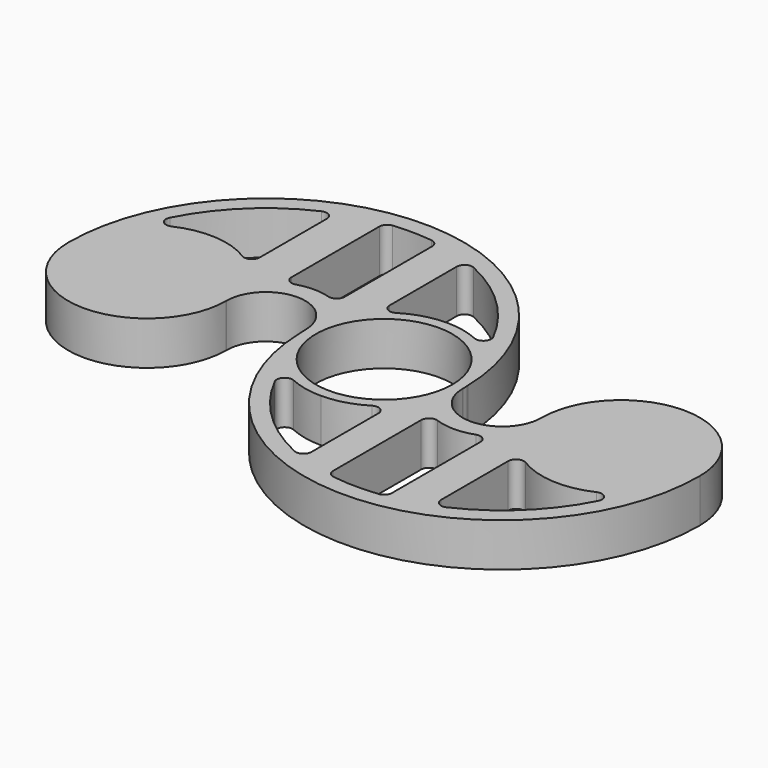
from build123d import *

# Parameters (mm, degrees)
F0_R        = 10.9855
F0_R_2      = 10.989999991
F1_DEPTH    = 7
F2_T1_DEPTH = 7
F2_T3_DEPTH = 7.1579854221
F2_T5_DEPTH = 7.1579856015
F2_T7_DEPTH = 7.1579856772
F3_R        = 1.27


# Not quite as in the source:
# - a fillet or chamfer that OpenCascade refuses, or shapes differently, is made with other operations: its cross-section is extruded or revolved along the edge and cut away or added
# - a feature names something its author has since deleted; it is built from what else it names


with BuildPart() as f1:
    # F0 (on Top) → F1 (new body)
    with BuildSketch(Plane.XY):
        with BuildLine():
            ThreePointArc((0.0122500747, -12.699994092), (8.9845861326, -8.9759240207), (12.7, 0))
            ThreePointArc((12.7, 0), (11.6341942626, 5.0926931834), (8.6156655339, 9.3306113095))
            ThreePointArc((8.6156655339, 9.3306113095), (4.6312435718, 11.8254633304), (0.0122500747, 12.699994092))
            ThreePointArc((0.0122500747, 12.699994092), (-4.6067434223, 11.8254633304), (-8.5911653844, 9.3306113095))
            ThreePointArc((-8.5911653844, 9.3306113095), (-11.6096941131, 5.0926931834), (-12.6754998505, 0))
            ThreePointArc((-12.6754998505, 0), (-11.6096941131, -5.0926931834), (-8.5911653844, -9.3306113095))
            ThreePointArc((-8.5911653844, -9.3306113095), (-4.6067434223, -11.8254633304), (0.0122500747, -12.699994092))
        make_face()
        with Locations((0.0245001495, 0)):
            Circle(F0_R, mode=Mode.SUBTRACT)
        with BuildLine():
            ThreePointArc((12.7245001495, 0), (12.716207726, 0.4588668575), (12.6913412845, 0.9171344838))
            ThreePointArc((12.6913412845, 0.9171344838), (12.6989837582, 0.4585985212), (12.7, 0))
            ThreePointArc((12.7, 0), (8.9845861326, -8.9759240207), (0.0122500747, -12.699994092))
            ThreePointArc((0.0122500747, -12.699994092), (4.6443350463, -11.8299250009), (8.6401656833, -9.3306113095))
            ThreePointArc((8.6401656833, -9.3306113095), (10.2086695664, -7.5876671836), (11.4300151579, -5.586074417))
            ThreePointArc((11.4300151579, -5.586074417), (12.3868415398, -2.9090402797), (12.7242073512, -0.086237983))
            ThreePointArc((12.7242073512, -0.086237983), (12.7242070748, -0.0431184935), (12.7245001495, 0))
        make_face()
        with BuildLine():
            ThreePointArc((25.4002735579, -0.086237983), (19.0622404546, -6.4027075191), (12.7242073512, -0.086237983))
            ThreePointArc((12.7242073512, -0.086237983), (12.3868415398, -2.9090402797), (11.4300151579, -5.586074417))
            ThreePointArc((11.4300151579, -5.586074417), (12.5867658694, -6.9038365057), (13.9769937331, -7.9724035921))
            ThreePointArc((13.9769937331, -7.9724035921), (18.7426985376, -9.3370960194), (23.5084033421, -7.9724035921))
            ThreePointArc((23.5084033421, -7.9724035921), (25.1435205419, -6.6655071902), (26.4326717576, -5.0163632895))
            ThreePointArc((26.4326717576, -5.0163632895), (25.6695984826, -2.6029975888), (25.4002735579, -0.086237983))
        make_face()
        with BuildLine():
            ThreePointArc((46.7156462935, -9.3306113095), (49.7341750222, -5.0926931834), (50.7999807596, 0))
            ThreePointArc((50.7999807596, 0), (38.0999807596, 12.7), (25.3999807596, 0))
            ThreePointArc((25.3999807596, 0), (25.4002738343, -0.0431184935), (25.4002735579, -0.086237983))
            ThreePointArc((25.4002735579, -0.086237983), (25.6695984826, -2.6029975888), (26.4326717576, -5.0163632895))
            ThreePointArc((26.4326717576, -5.0163632895), (27.7316179187, -7.3339656394), (29.4843152258, -9.3306113095))
            ThreePointArc((29.4843152258, -9.3306113095), (38.0999807596, -12.7), (46.7156462935, -9.3306113095))
        make_face()
        with Locations((38.0999807596, 0)):
            Circle(F0_R_2, mode=Mode.SUBTRACT)
        with BuildLine():
            ThreePointArc((-8.5801649897, -9.3632669913), (-11.43210855, -5.5314459322), (-12.666841135, -0.9171344838))
            ThreePointArc((-12.666841135, -0.9171344838), (19.5208281328, -31.8937955885), (50.7999807596, 0))
            ThreePointArc((50.7999807596, 0), (49.7341750222, -5.0926931834), (46.7156462935, -9.3306113095))
            ThreePointArc((46.7156462935, -9.3306113095), (40.1099512813, -20.2359805679), (29.4843152258, -27.2828340268))
            ThreePointArc((29.4843152258, -27.2828340268), (26.5384433366, -28.2337157759), (23.5084033421, -28.8671152702))
            ThreePointArc((23.5084033421, -28.8671152702), (18.7383474141, -29.2061036376), (13.9769937331, -28.7612915499))
            ThreePointArc((13.9769937331, -28.7612915499), (11.2734206382, -28.1489774328), (8.6401656833, -27.2828340268))
            ThreePointArc((8.6401656833, -27.2828340268), (-1.9735358373, -20.2484070502), (-8.5801649897, -9.3632669913))
        make_face()
        with BuildLine():
            ThreePointArc((-11.4055150084, 5.586074417), (-12.3623413903, 2.9090402797), (-12.6997072018, 0.086237983))
            ThreePointArc((-12.6997072018, 0.086237983), (-12.6997069253, 0.0431184935), (-12.7, 0))
            ThreePointArc((-12.7, 0), (-12.6917075765, -0.4588668575), (-12.666841135, -0.9171344838))
            ThreePointArc((-12.666841135, -0.9171344838), (-12.6744836087, -0.4585985212), (-12.6754998505, 0))
            ThreePointArc((-12.6754998505, 0), (-11.6096941131, 5.0926931834), (-8.5911653844, 9.3306113095))
            Line((-8.5911653844, 9.3306113095), (-8.5911653844, 9.3531747198))
            ThreePointArc((-8.5911653844, 9.3531747198), (-10.1742109205, 7.6010152049), (-11.4055150084, 5.586074417))
        make_face()
        with BuildLine():
            ThreePointArc((-22.9900462212, 8.2591606127), (-24.9149898439, 6.8653148973), (-26.4081716081, 5.0163632895))
            ThreePointArc((-26.4081716081, 5.0163632895), (-25.6450983331, 2.6029975888), (-25.3757734084, 0.086237983))
            ThreePointArc((-25.3757734084, 0.086237983), (-19.0377403051, 6.4027075191), (-12.6997072018, 0.086237983))
            ThreePointArc((-12.6997072018, 0.086237983), (-12.3623413903, 2.9090402797), (-11.4055150084, 5.586074417))
            ThreePointArc((-11.4055150084, 5.586074417), (-12.773731355, 7.0957580254), (-14.446350555, 8.2591606127))
            ThreePointArc((-14.446350555, 8.2591606127), (-18.7181983881, 9.3370960194), (-22.9900462212, 8.2591606127))
        make_face()
        with BuildLine():
            ThreePointArc((-25.3757734084, 0.086237983), (-25.6450983331, 2.6029975888), (-26.4081716081, 5.0163632895))
            ThreePointArc((-26.4081716081, 5.0163632895), (-27.7071177693, 7.3339656394), (-29.4598150763, 9.3306113095))
            ThreePointArc((-29.4598150763, 9.3306113095), (-38.0754806101, 12.7), (-46.691146144, 9.3306113095))
            ThreePointArc((-46.691146144, 9.3306113095), (-49.7096748727, 5.0926931834), (-50.7754806101, 0))
            ThreePointArc((-50.7754806101, 0), (-38.0754806101, -12.7), (-25.3754806101, 0))
            ThreePointArc((-25.3754806101, 0), (-25.3757736848, 0.0431184935), (-25.3757734084, 0.086237983))
        make_face()
        with Locations((-38.0754806101, 0)):
            Circle(F0_R_2, mode=Mode.SUBTRACT)
        with BuildLine():
            ThreePointArc((-8.5911653844, -9.3306113095), (-8.5856700083, -9.3469407745), (-8.5801649897, -9.3632669913))
            ThreePointArc((-8.5801649897, -9.3632669913), (-4.5973610293, -11.8386769348), (0.0122500747, -12.699994092))
            ThreePointArc((0.0122500747, -12.699994092), (-4.6067434223, -11.8254633304), (-8.5911653844, -9.3306113095))
        make_face()
        with BuildLine():
            ThreePointArc((-12.6754998505, 0), (-12.6744836087, -0.4585985212), (-12.666841135, -0.9171344838))
            ThreePointArc((-12.666841135, -0.9171344838), (-11.43210855, -5.5314459322), (-8.5801649897, -9.3632669913))
            ThreePointArc((-8.5801649897, -9.3632669913), (-8.5856700083, -9.3469407745), (-8.5911653844, -9.3306113095))
            ThreePointArc((-8.5911653844, -9.3306113095), (-11.6096941131, -5.0926931834), (-12.6754998505, 0))
        make_face()
        with BuildLine():
            ThreePointArc((12.7, 0), (12.6989837582, 0.4585985212), (12.6913412845, 0.9171344838))
            ThreePointArc((12.6913412845, 0.9171344838), (11.4566086995, 5.5314459323), (8.6046651392, 9.3632669913))
            ThreePointArc((8.6046651392, 9.3632669913), (8.6101701578, 9.3469407745), (8.6156655339, 9.3306113095))
            ThreePointArc((8.6156655339, 9.3306113095), (11.6341942626, 5.0926931834), (12.7, 0))
        make_face()
        with BuildLine():
            ThreePointArc((8.6156655339, 9.3306113095), (8.6101701578, 9.3469407745), (8.6046651392, 9.3632669913))
            ThreePointArc((8.6046651392, 9.3632669913), (4.6218611788, 11.8386769348), (0.0122500747, 12.699994092))
            ThreePointArc((0.0122500747, 12.699994092), (4.6312435718, 11.8254633304), (8.6156655339, 9.3306113095))
        make_face()
        with BuildLine():
            ThreePointArc((-50.7754806101, 0), (-49.7096748727, 5.0926931834), (-46.691146144, 9.3306113095))
            ThreePointArc((-46.691146144, 9.3306113095), (-40.0854511318, 20.2359805679), (-29.4598150763, 27.2828340268))
            ThreePointArc((-29.4598150763, 27.2828340268), (-26.2724748955, 28.2966277505), (-22.9900462212, 28.9389494304))
            ThreePointArc((-22.9900462212, 28.9389494304), (-18.7147163655, 29.2061132739), (-14.446350555, 28.8443464952))
            ThreePointArc((-14.446350555, 28.8443464952), (-11.4778445606, 28.2113948339), (-8.5911653844, 27.2734508175))
            ThreePointArc((-8.5911653844, 27.2734508175), (2.0071231414, 20.238946653), (8.6046651392, 9.3632669913))
            ThreePointArc((8.6046651392, 9.3632669913), (11.4566086995, 5.5314459323), (12.6913412845, 0.9171344838))
            ThreePointArc((12.6913412845, 0.9171344838), (-19.4963279834, 31.8937955885), (-50.7754806101, 0))
        make_face()
        with BuildLine():
            Line((-14.446350555, 28.8443464952), (-14.446350555, 8.2591606127))
            ThreePointArc((-14.446350555, 8.2591606127), (-12.773731355, 7.0957580254), (-11.4055150084, 5.586074417))
            ThreePointArc((-11.4055150084, 5.586074417), (-10.1742109205, 7.6010152049), (-8.5911653844, 9.3531747198))
            Line((-8.5911653844, 9.3531747198), (-8.5911653844, 27.2734508175))
            ThreePointArc((-8.5911653844, 27.2734508175), (-11.4778445606, 28.2113948339), (-14.446350555, 28.8443464952))
        make_face()
        with BuildLine():
            ThreePointArc((-29.4598150763, 9.3306113095), (-27.7071177693, 7.3339656394), (-26.4081716081, 5.0163632895))
            ThreePointArc((-26.4081716081, 5.0163632895), (-24.9149898439, 6.8653148973), (-22.9900462212, 8.2591606127))
            Line((-22.9900462212, 8.2591606127), (-22.9900462212, 28.9389494304))
            ThreePointArc((-22.9900462212, 28.9389494304), (-26.2724748955, 28.2966277505), (-29.4598150763, 27.2828340268))
            Line((-29.4598150763, 27.2828340268), (-29.4598150763, 9.3306113095))
        make_face()
        with BuildLine():
            Line((8.6401656833, -9.3306113095), (8.6401656833, -27.2828340268))
            ThreePointArc((8.6401656833, -27.2828340268), (11.2734206382, -28.1489774328), (13.9769937331, -28.7612915499))
            Line((13.9769937331, -28.7612915499), (13.9769937331, -7.9724035921))
            ThreePointArc((13.9769937331, -7.9724035921), (12.5867658694, -6.9038365057), (11.4300151579, -5.586074417))
            ThreePointArc((11.4300151579, -5.586074417), (10.2086695664, -7.5876671836), (8.6401656833, -9.3306113095))
        make_face()
        with BuildLine():
            Line((29.4843152258, -27.2828340268), (29.4843152258, -9.3306113095))
            ThreePointArc((29.4843152258, -9.3306113095), (27.7316179187, -7.3339656394), (26.4326717576, -5.0163632895))
            ThreePointArc((26.4326717576, -5.0163632895), (25.1435205419, -6.6655071902), (23.5084033421, -7.9724035921))
            Line((23.5084033421, -7.9724035921), (23.5084033421, -28.8671152702))
            ThreePointArc((23.5084033421, -28.8671152702), (26.5384433366, -28.2337157759), (29.4843152258, -27.2828340268))
        make_face()
        with Locations((-38.0754806101, 0)):
            Circle(F0_R_2)
        with Locations((38.0999807596, 0)):
            Circle(F0_R_2)
    extrude(amount=F1_DEPTH)

    # F2: fillet of radius 5.08 on 9 edges, made by hand

    # F2_s2 → F2_t1 (join)
    with BuildSketch(Plane.XY):
        with BuildLine():
            ThreePointArc((-50.7755312412, 0.0104518732), (-50.7754943345, 0.0004688293), (-50.7754770463, -0.0095142678))
            ThreePointArc((-50.7754770463, -0.0095142678), (-50.7754797192, -0.0047571342), (-50.7754806101, 0))
            ThreePointArc((-50.7754806101, 0), (-50.7755063559, 0.0052259345), (-50.7755312412, 0.0104518732))
        make_face()
        with BuildLine():
            ThreePointArc((-12.6731476592, -0.8254261976), (-12.6677935321, -0.9217143052), (-12.6642681854, -1.018086699))
            ThreePointArc((-12.6642681854, -1.018086699), (-12.6655948117, -0.9676116147), (-12.666841135, -0.9171344838))
            ThreePointArc((-12.666841135, -0.9171344838), (-12.6700773725, -0.8712860467), (-12.6731476592, -0.8254261976))
        make_face()
        with BuildLine():
            ThreePointArc((12.6976478087, 0.8254261976), (12.6922936816, 0.9217143052), (12.6887683349, 1.018086699))
            ThreePointArc((12.6887683349, 1.018086699), (12.6900949612, 0.9676116147), (12.6913412845, 0.9171344838))
            ThreePointArc((12.6913412845, 0.9171344838), (12.694577522, 0.8712860467), (12.6976478087, 0.8254261976))
        make_face()
        with BuildLine():
            ThreePointArc((50.8000313907, -0.0104518732), (50.799994484, -0.0004688294), (50.7999771958, 0.0095142678))
            ThreePointArc((50.7999771958, 0.0095142678), (50.7999798687, 0.0047571342), (50.7999807596, 0))
            ThreePointArc((50.7999807596, 0), (50.8000065054, -0.0052259345), (50.8000313907, -0.0104518732))
        make_face()
    extrude(amount=F2_T1_DEPTH)

    # F2_s4 → F2_t3 (cut)
    with BuildSketch(Plane.XY.offset(-0.0789927111)):
        with BuildLine():
            ThreePointArc((-12.6998402645, 0.0182342924), (-12.6999615812, -0.0066812361), (-12.6999606939, -0.03159706))
            ThreePointArc((-12.6999606939, -0.03159706), (-12.6999901735, -0.0157985422), (-12.7, 0))
            ThreePointArc((-12.7, 0), (-12.6999135747, 0.0091170887), (-12.6998402645, 0.0182342924))
        make_face()
    extrude(amount=F2_T3_DEPTH, mode=Mode.SUBTRACT)

    # F2_s6 → F2_t5 (cut)
    with BuildSketch(Plane.XY.offset(-0.0789928007)):
        with BuildLine():
            ThreePointArc((-25.3756403458, 0.0182342804), (-25.375519029, -0.0066812601), (-25.3755199164, -0.0315970958))
            ThreePointArc((-25.3755199164, -0.0315970958), (-25.3754904367, -0.0157985601), (-25.3754806101, 0))
            ThreePointArc((-25.3754806101, 0), (-25.3755670356, 0.0091170828), (-25.3756403458, 0.0182342804))
        make_face()
        with BuildLine():
            ThreePointArc((25.4000200658, 0.0315970958), (25.4000191785, 0.0066812601), (25.4001404953, -0.0182342804))
            ThreePointArc((25.4001404953, -0.0182342804), (25.4000671851, -0.0091170828), (25.3999807596, 0))
            ThreePointArc((25.3999807596, 0), (25.3999905862, 0.0157985601), (25.4000200658, 0.0315970958))
        make_face()
    extrude(amount=F2_T5_DEPTH, mode=Mode.SUBTRACT)

    # F2_s8 → F2_t7 (cut)
    with BuildSketch(Plane.XY.offset(-0.0789928386)):
        with BuildLine():
            ThreePointArc((12.7243404138, -0.0182342754), (12.7244617306, 0.0066812701), (12.7244608432, 0.031597111))
            ThreePointArc((12.7244608432, 0.031597111), (12.7244903229, 0.0157985677), (12.7245001495, 0))
            ThreePointArc((12.7245001495, 0), (12.724413724, -0.0091170802), (12.7243404138, -0.0182342754))
        make_face()
    extrude(amount=F2_T7_DEPTH, mode=Mode.SUBTRACT)

    # F3
    f3_edges = [f1.edges().sort_by_distance(p)[0] for p in [
        (29.484315, -27.282834, 3.5),
        (29.484315, -9.330611, 3.5),
        (46.715646, -9.330611, 3.5),
        (23.508403, -7.972404, 3.5),
        (13.976994, -7.972404, 3.5),
        (23.508403, -28.867115, 3.5),
        (13.976994, -28.761292, 3.5),
        (8.640166, -27.282834, 3.5),
        (8.640166, -9.330611, 3.5),
        (-8.580165, -9.363267, 3.5),
        (-22.990046, 28.938949, 3.5),
        (-8.591165, 27.273451, 3.5),
        (8.604665, 9.363267, 3.5),
        (-8.591165, 9.330611, 3.5),
        (-22.990046, 8.259161, 3.5),
        (-14.446351, 8.259161, 3.5),
        (-14.446351, 28.844346, 3.5),
        (-29.459815, 9.330611, 3.5),
        (-29.459815, 27.282834, 3.5),
        (-46.691146, 9.330611, 3.5),
    ]]
    fillet(f3_edges, radius=F3_R)


solid = f1.part
